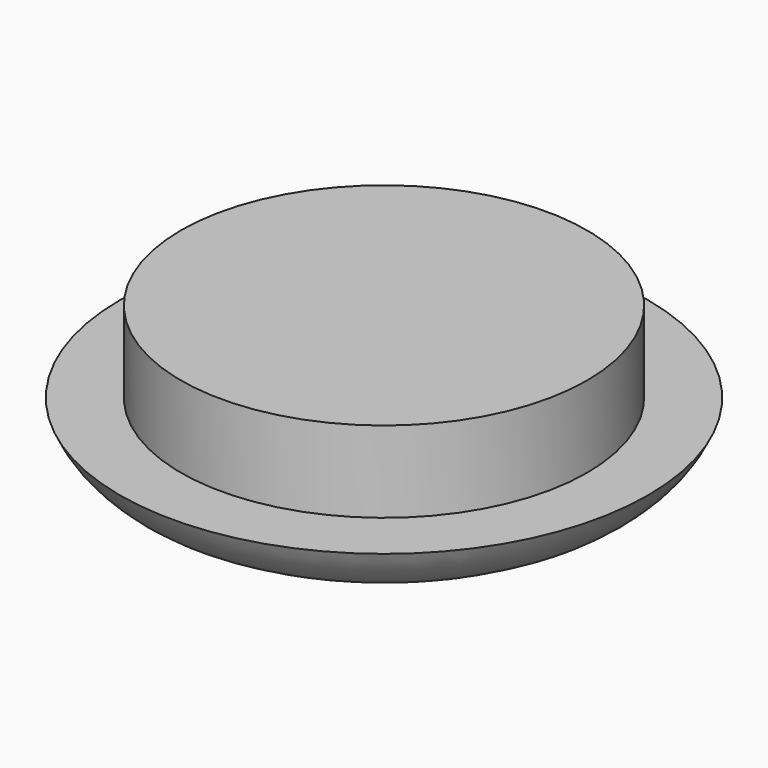
from build123d import *

# Parameters (mm, degrees)
F1_R     = 10
F2_DEPTH = 7
F0_R     = 13
F3_DEPTH = 3


# Not quite as in the source:
# - a fillet or chamfer that OpenCascade refuses, or shapes differently, is made with other operations: its cross-section is extruded or revolved along the edge and cut away or added


with BuildPart() as f2:
    # F1 (on Top) → F2 (new body)
    with BuildSketch(Plane.XY):
        Circle(F1_R)
    extrude(amount=F2_DEPTH)

    # F0 (on Top) → F3 (join)
    with BuildSketch(Plane.XY):
        Circle(F0_R)
    extrude(amount=F3_DEPTH)

    # F4: fillet of radius 5 on 1 edges, made by hand

    # F4_s1 → F4_t2 (revolve, cut)
    with BuildSketch(Plane.XZ):
        with BuildLine():
            ThreePointArc((8.417424305, 0), (11.1560370926, 0.8166998673), (13, 3))
            Line((13, 3), (13, 0))
            Line((13, 0), (8.417424305, 0))
        make_face()
    revolve(axis=Axis((0, 0, 0), (0, 0, 1)), mode=Mode.SUBTRACT)


solid = f2.part
